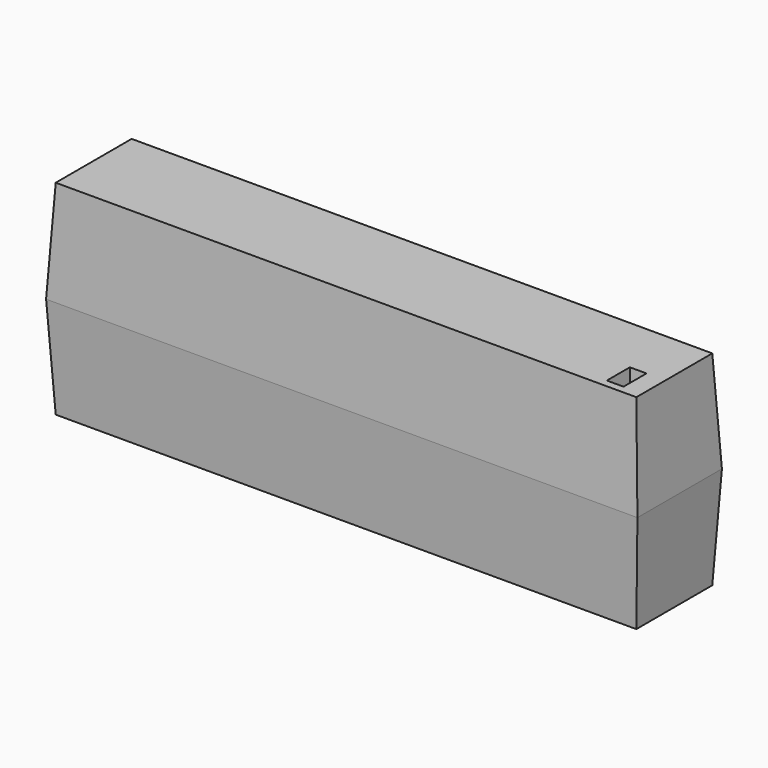
from build123d import *

# Parameters (mm, degrees)
F0_W     = 0.7410570979
F0_H     = 2.2417232394
F1_DEPTH = 12.7
F1_TAPER = 3


with BuildPart() as f1:
    # F0 (on Top) → F1 (new body, symmetric)
    with BuildSketch(Plane.XY):
        Polygon((65.8400952816, 61.8246868253), (73.5567137599, 61.8246868253), (73.5567137599, 74.9637633562), (0, 74.9637633562), (0, 61.8246868253), align=None)
        with Locations((69.5021115243, 65.2226097882)):
            Rectangle(F0_W, F0_H, mode=Mode.SUBTRACT)
    extrude(amount=F1_DEPTH, both=True, taper=F1_TAPER)


solid = f1.part
